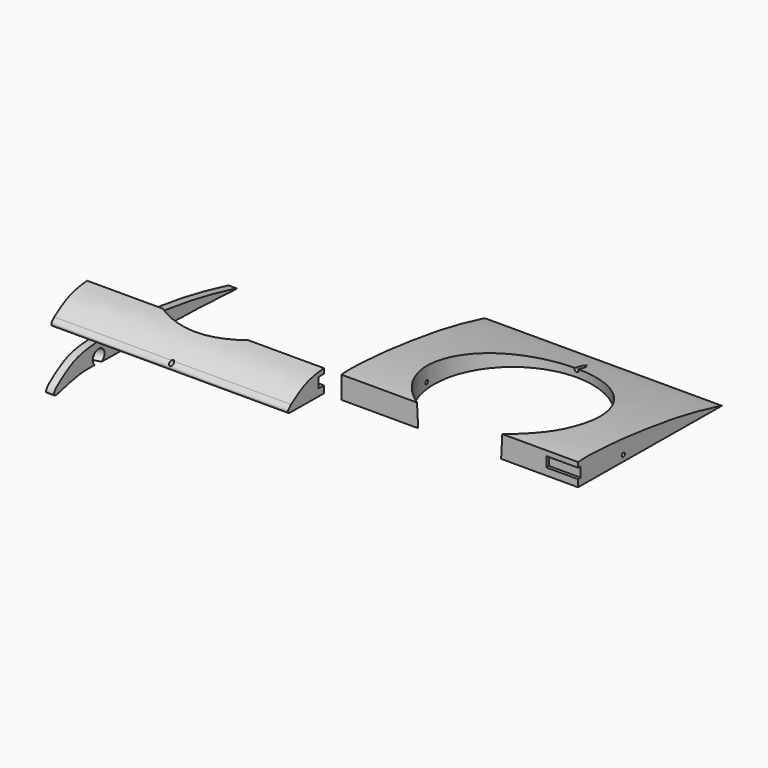
from build123d import *

# Parameters (mm, degrees)
F1_DEPTH       = 5
F4_R           = 4.4
F5_DEPTH       = 25
F5_DEPTH_BACK  = 25
F7_DEPTH       = 150
F10_R          = 50
F11_DEPTH      = 79
F15_R          = 1.25
F18_DEPTH      = 81
F18_DEPTH_BACK = 95
F17_R          = 1.25
F19_DEPTH      = 79.7
F19_DEPTH_BACK = 89.9
F20_W          = 6.4
F20_H          = 6.4
F21_DEPTH      = 20
F22_W          = 6.4
F22_H          = 6.4
F22_R          = 1.284850819
F23_DEPTH      = 20
F25_W          = 166.2742132321
F25_H          = 124.5705988258
F26_DEPTH      = 80
F25_W_2        = 196.187093854
F25_H_2        = 51.8369693309
F27_DEPTH      = 80


with BuildPart() as f1:
    # F0 (on Right) → F1 (new body)
    with BuildSketch(Plane.YZ):
        with BuildLine():
            add(Edge.make_bspline(
                [(-58.3274115764, -12.0050430576), (-58.3344388652, -11.4569577771), (-57.6057042665, -9.7696015427), (-53.3968805544, -6.2080779669), (-43.9658631609, -0.1790497745), (-35.1048713842, 2.4961867136), (-21.2595411738, 3.8461410587), (-5.824125135, 2.6266429273), (5.6371044072, 2.1477470473), (30.3775327494, -0.7795886798), (56.2487237073, -4.4526809054), (81.8846479865, -10.4041940314), (87.5956539626, -12.0042825946), (82.9344545505, -11.7909369576), (69.2602600576, -11.0597506918), (43.6004036943, -10.0115889059), (9.9369455047, -9.4817909084), (-11.6934189582, -9.1940065774), (-19.9470741332, -9.2146394297), (-24.1603477555, -8.9849455596), (-24.9304296118, -8.9420522318)],
                knots=[0, 0, 0, 0, 0.0187688844, 0.0496730335, 0.0939697776, 0.1345871316, 0.1839900585, 0.2358076841, 0.2809157421, 0.3457702283, 0.4171824372, 0.4853410136, 0.5086588268, 0.5293900877, 0.5781157074, 0.6466821194, 0.7250191339, 0.7862544333, 0.8291256087, 0.838576028, 0.838576028, 0.838576028, 0.838576028], degree=3))
            add(Edge.make_bspline(
                [(-28.5969946171, -8.7548278676), (-30.207848663, -8.6901905412), (-35.3665317632, -8.5989901045), (-43.4073330182, -9.9616339771), (-51.553031371, -11.8830223488), (-57.7998585373, -13.5752431948), (-58.3222069698, -12.4109703396), (-58.3274115764, -12.0050430576)],
                knots=[0.8533695632, 0.8533695632, 0.8533695632, 0.8533695632, 0.8726905599, 0.914874294, 0.954646186, 0.9860992395, 1, 1, 1, 1], degree=3))
            add(Edge.make_bspline(
                [(-24.9304296118, -8.9420522318), (-26.135903424, -8.8749077029), (-27.3636097023, -8.8043188214), (-28.5969946171, -8.7548278676)],
                knots=[0.838576028, 0.838576028, 0.838576028, 0.838576028, 0.8533695632, 0.8533695632, 0.8533695632, 0.8533695632], degree=3))
        make_face()
        with BuildLine():
            Line((-28.5969946171, -8.7548278676), (-24.9304296118, -8.9420522318))
            add(Edge.make_bspline(
                [(-24.9304296118, -8.9420522318), (-26.135903424, -8.8749077029), (-27.3636097023, -8.8043188214), (-28.5969946171, -8.7548278676)],
                knots=[0.838576028, 0.838576028, 0.838576028, 0.838576028, 0.8533695632, 0.8533695632, 0.8533695632, 0.8533695632], degree=3))
        make_face()
    extrude(amount=F1_DEPTH)

    # F4 (on line) → F5 (cut, two sides)
    with BuildSketch(Plane(origin=(-2.2217460192, -0.8086414928, 0), x_dir=(0.342017183, -0.9396936982, 0), z_dir=(-0.9396936982, -0.342017183, 0))) as f5_sk:
        with Locations((23.2877507806, -5.3645325825)):
            Circle(F4_R)
    extrude(amount=-F5_DEPTH, mode=Mode.SUBTRACT)
    extrude(f5_sk.sketch, amount=F5_DEPTH_BACK, mode=Mode.SUBTRACT)


with BuildPart() as f7:
    # F6 (on Right) → F7 (new body)
    with BuildSketch(Plane.YZ):
        with BuildLine():
            Line((85.249999757, 21.6100029291), (88.1275390807, 21.5883248069))
            add(Edge.make_bspline(
                [(-51.882735866, 26.8891940408), (-49.2317247895, 28.8257538777), (-42.3172155877, 33.2460374139), (-33.456223811, 35.9212739021), (-19.6108936006, 37.2712282472), (-4.1754775618, 36.0517301158), (7.2857519804, 35.5728342357), (32.0261803226, 32.6454985086), (57.8973712806, 28.972406283), (83.5332955597, 23.0208931571), (88.1891475039, 21.7164337538), (88.1275390807, 21.5883248069)],
                knots=[0.0496730335, 0.0496730335, 0.0496730335, 0.0496730335, 0.0939697776, 0.1345871316, 0.1839900585, 0.2358076841, 0.2809157421, 0.3457702283, 0.4171824372, 0.4853410136, 0.5086588268, 0.5086588268, 0.5086588268, 0.5086588268], degree=3))
            add(Edge.make_bspline(
                [(-51.882735866, 26.8891940408), (-52.8135655, 26.0844658354), (-54.3176059268, 24.7841808913), (-54.1871855038, 23.2740306963), (-53.7061726576, 22.8500568138), (-53.4850694242, 22.6551722372)],
                knots=[0, 0, 0, 0, 0.4673621583, 0.7551667333, 1, 1, 1, 1], degree=3))
            Line((-53.4850694242, 22.6551722372), (-45.3372013165, 22.5937897639))
            add(Edge.make_bspline(
                [(85.249999757, 21.6100029291), (82.0924248153, 21.7672634923), (70.6206337647, 22.3771119972), (45.2490512675, 23.4134982826), (11.5855930779, 23.94329628), (-10.044771385, 24.231080611), (-20.7779729143, 24.2042492791), (-31.7930488816, 25.1522915708), (-39.8664798, 23.7841180737), (-44.1691237236, 22.8583410653), (-45.3372013165, 22.5937897639)],
                knots=[0.5315878686, 0.5315878686, 0.5315878686, 0.5315878686, 0.5781157074, 0.6466821194, 0.7250191339, 0.7862544333, 0.8291256087, 0.8726905599, 0.914874294, 0.9308132132, 0.9308132132, 0.9308132132, 0.9308132132], degree=3))
        make_face()
        with BuildLine():
            Line((-45.3372013165, 22.5937897639), (85.249999757, 21.6100029291))
            add(Edge.make_bspline(
                [(85.249999757, 21.6100029291), (82.0924248153, 21.7672634923), (70.6206337647, 22.3771119972), (45.2490512675, 23.4134982826), (11.5855930779, 23.94329628), (-10.044771385, 24.231080611), (-20.7779729143, 24.2042492791), (-31.7930488816, 25.1522915708), (-39.8664798, 23.7841180737), (-44.1691237236, 22.8583410653), (-45.3372013165, 22.5937897639)],
                knots=[0.5315878686, 0.5315878686, 0.5315878686, 0.5315878686, 0.5781157074, 0.6466821194, 0.7250191339, 0.7862544333, 0.8291256087, 0.8726905599, 0.914874294, 0.9308132132, 0.9308132132, 0.9308132132, 0.9308132132], degree=3))
        make_face()
    extrude(amount=F7_DEPTH)

    # F10 (on line) → F11 (cut)
    with BuildSketch(Plane(origin=(0, -2.436713941, 73.1014182314), x_dir=(1, 0, 0), z_dir=(0, -0.0333148302, 0.999444907))):
        with Locations((75, 17.4860656261)):
            Circle(F10_R)
    extrude(amount=-F11_DEPTH, mode=Mode.SUBTRACT)

    # F15 (on plane+point) → F18 (cut, two sides)
    with BuildSketch(Plane.YZ.offset(75.1169547439)) as f18_sk:
        with Locations((10.0469859317, 25.9796357161)):
            Circle(F15_R)
    extrude(amount=-F18_DEPTH, mode=Mode.SUBTRACT)
    extrude(f18_sk.sketch, amount=F18_DEPTH_BACK, mode=Mode.SUBTRACT)

    # F17 (on plane+point) → F19 (cut, two sides)
    with BuildSketch(Plane.XZ.offset(-10.0469859317)) as f19_sk:
        with Locations((75.1169547439, 25.9796357161)):
            Circle(F17_R)
    extrude(amount=-F19_DEPTH, mode=Mode.SUBTRACT)
    extrude(f19_sk.sketch, amount=F19_DEPTH_BACK, mode=Mode.SUBTRACT)

    # F20 (on face) → F21 (cut)
    with BuildSketch(Plane.YZ.offset(150)):
        with Locations((-26.8901380122, 30.1654917777)):
            Rectangle(F20_W, F20_H)
    extrude(amount=-F21_DEPTH, mode=Mode.SUBTRACT)

    # F22 (on face) → F23 (cut)
    with BuildSketch(Plane(origin=(0, 0, 0), x_dir=(0, -1, 0), z_dir=(-1, 0, 0))):
        with Locations((0.7321151562, 29.7433977604)):
            Rectangle(F22_W, F22_H)
        with Locations((-63.4693279862, 24.8407572508)):
            Circle(F22_R)
        with Locations((31.9451669574, 29.525289464)):
            Rectangle(F22_W, F22_H)
    extrude(amount=-F23_DEPTH, mode=Mode.SUBTRACT)


with BuildPart() as f24_1:
    # F24: copy of F7
    add(f7.part.moved(Location((161, 0, 0))))

    # F25 (on Top) → F27 (cut)
    with BuildSketch(Plane.XY):
        with Locations((252.154968679, -51.7409509048)):
            Rectangle(F25_W_2, F25_H_2)
    extrude(amount=F27_DEPTH, mode=Mode.SUBTRACT)


with BuildPart() as f7_1:
    add(f7.part)

    # F25 (on Top) → F26 (cut)
    with BuildSketch(Plane.XY):
        with Locations((70.9243151359, 36.4628331736)):
            Rectangle(F25_W, F25_H)
    extrude(amount=F26_DEPTH, mode=Mode.SUBTRACT)


solid = Compound([f1.part, f24_1.part, f7_1.part])
